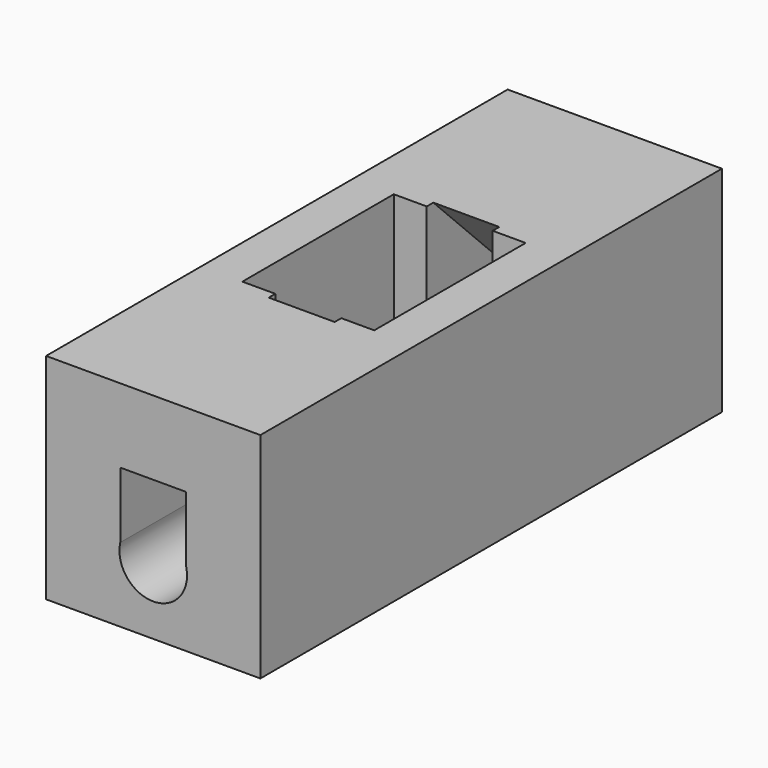
from build123d import *

# Parameters (mm, degrees)
F0_W        = 2.6
F0_H        = 2.6
F1_DEPTH    = 7
F2_W        = 1.6
F2_H        = 2.2962607759
F3_DEPTH    = 25
F4_T1_DEPTH = 0.8


# Not quite as in the source:
# - a fillet or chamfer that OpenCascade refuses, or shapes differently, is made with other operations: its cross-section is extruded or revolved along the edge and cut away or added


with BuildPart() as f1:
    # F0 (on Front) → F1 (new body)
    with BuildSketch(Plane.XZ):
        with Locations((2.5521775242, -2.0290124111)):
            Rectangle(F0_W, F0_H)
        with BuildLine():
            Line((2.1521775242, -2.4290124111), (2.1521775242, -1.6290124111))
            Line((2.1521775242, -1.6290124111), (2.9521775242, -1.6290124111))
            Line((2.9521775242, -1.6290124111), (2.9521775242, -2.4290124111))
            ThreePointArc((2.9521775242, -2.4290124111), (2.9596698554, -2.4737354854), (2.9621775242, -2.5190124111))
            ThreePointArc((2.9621775242, -2.5190124111), (2.5069005985, -2.9265047423), (2.1521775242, -2.4290124111))
        make_face(mode=Mode.SUBTRACT)
    extrude(amount=F1_DEPTH)

    # F2 (on face) → F3 (cut)
    with BuildSketch(Plane(origin=(0, 0, -3.3290124111), x_dir=(1, 0, 0), z_dir=(0, 0, -1))):
        with Locations((2.5521775242, 3.5)):
            Rectangle(F2_W, F2_H)
    extrude(amount=-F3_DEPTH, mode=Mode.SUBTRACT)

    # F4: chamfer of 1 on 2 edges, made by hand

    # F4_s2 → F4_t1 (cut)
    with BuildSketch(Plane.YZ.offset(2.1521775242)):
        Polygon((-2.351869612, -0.6290124111), (-1.351869612, -1.6290124111), (-2.351869612, -1.6290124111), align=None)
        Polygon((-4.648130388, -0.6290124111), (-5.648130388, -1.6290124111), (-4.648130388, -1.6290124111), align=None)
    extrude(amount=F4_T1_DEPTH, mode=Mode.SUBTRACT)


solid = f1.part
